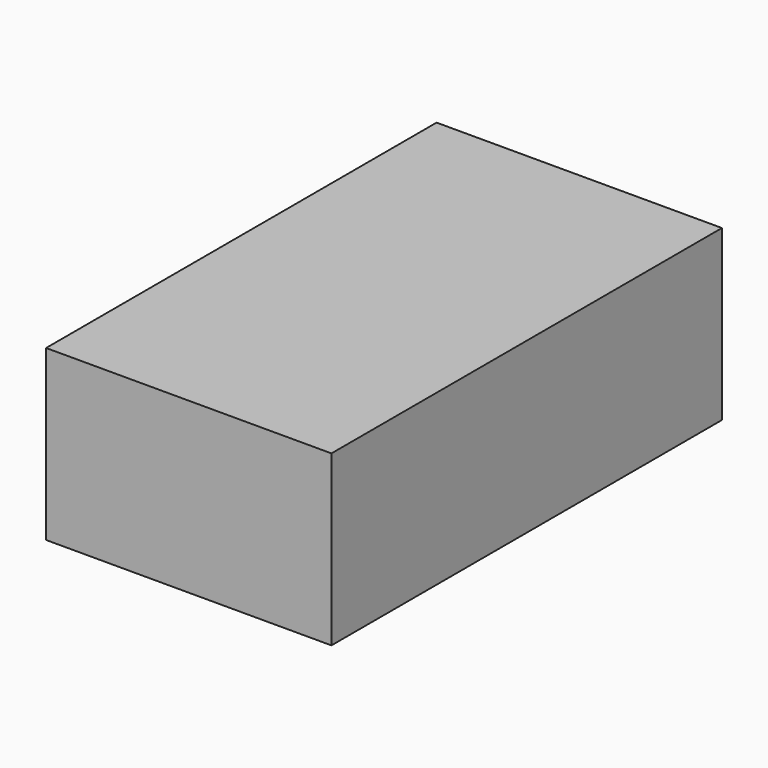
from build123d import *

# Parameters (mm, degrees)
F1_DEPTH = 63.5


# Not quite as in the source:
# - the program builds the solid bodies; features that only make, move or delete a surface that nothing else refers to are left out


with BuildPart() as f1:
    # F0 (on Front) → F1 (new body, symmetric)
    with BuildSketch(Plane.XZ):
        Polygon((-37.124483712, 21.9922941178), (-37.124483712, -21.9922941178), (37.124483712, -21.9922941178), (37.124483712, 21.9922941178), (0, 21.9922941178), (-11.9380000979, 21.9922941178), align=None)
    extrude(amount=F1_DEPTH, both=True)


solid = f1.part
